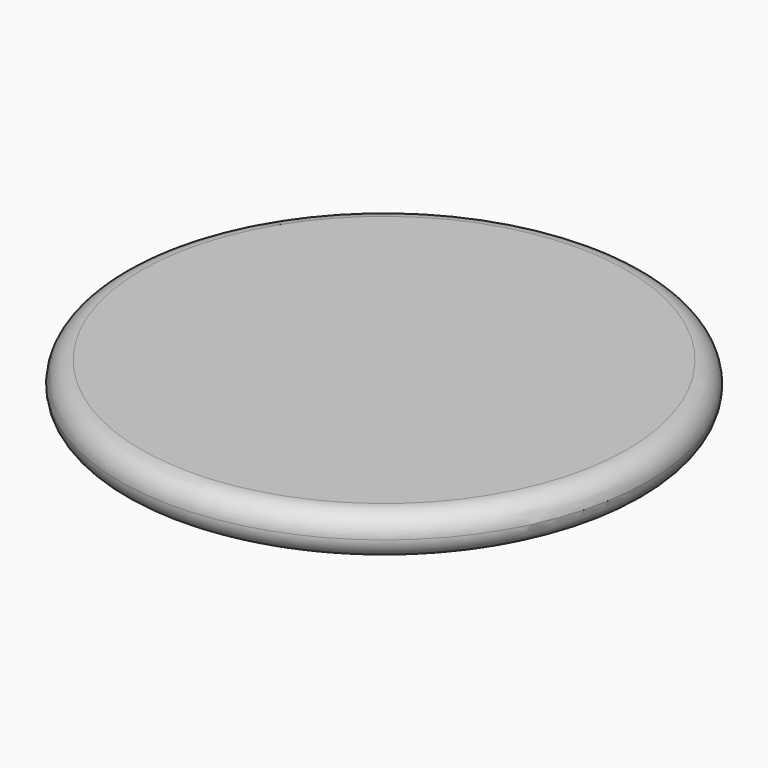
from build123d import *

# Parameters (mm, degrees)
F0_R     = 10
F1_DEPTH = 1.6
F2_R     = 0.79999


# Not quite as in the source:
# - a fillet or chamfer is up to 0.001 mm smaller than in the source, because OpenCascade refuses the exact size


with BuildPart() as f1:
    # F0 (on Top) → F1 (new body)
    with BuildSketch(Plane.XY):
        Circle(F0_R)
    extrude(amount=F1_DEPTH)

    # F2 (radius 0.8 in the source; OpenCascade refuses exactly that, so slightly less here)
    f2_edges = [f1.edges().sort_by_distance(p)[0] for p in [
        (-10, 0, 1.6),
        (-10, 0, 0),
    ]]
    fillet(f2_edges, radius=F2_R)


solid = f1.part
